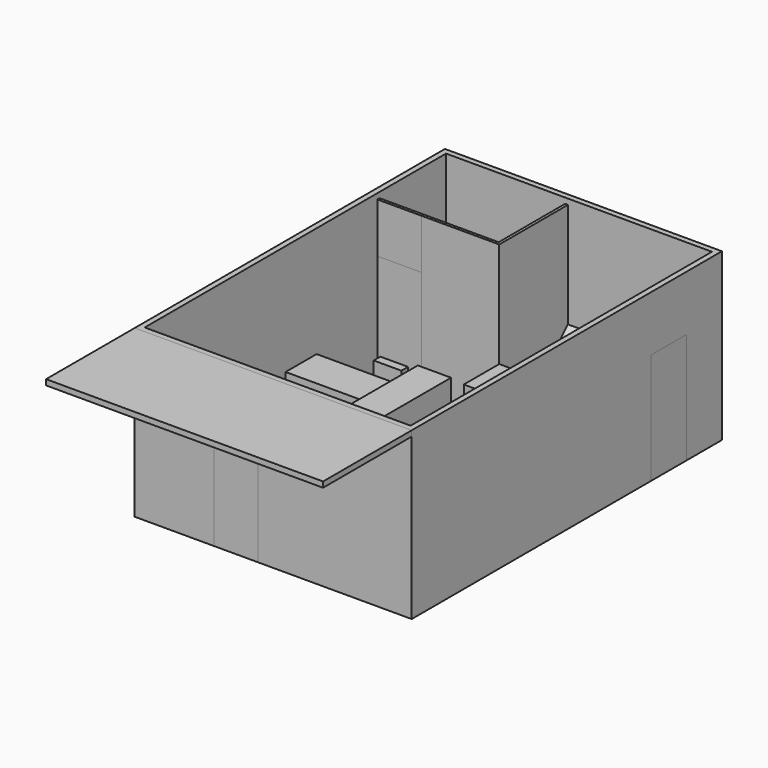
from build123d import *

# Parameters (mm, degrees)
F0_W      = 50
F0_H      = 70
F1_DEPTH  = 30
F2_T      = -1
F4_DEPTH  = 10
F3_W      = 4
F3_H      = 0.75
F3_W_2    = 5
F3_H_2    = 1.5
F3_H_3    = 5
F3_W_3    = 3
F3_H_4    = 3
F3_W_4    = 8.5
F3_H_5    = 3.5
F3_R      = 0.875
F5_DEPTH  = 6
F3_H_6    = 1.25
F3_H_7    = 18
F3_H_8    = 15
F6_DEPTH  = 20
F3_W_5    = 6.5
F3_W_6    = 0.2
F3_H_9    = 7
F3_H_10   = 8
F7_DEPTH  = 20
F8_DEPTH  = 10
F9_SIZE   = 9.99999
F10_DEPTH = 7
F12_DEPTH = 29
F3_W_7    = 8
F3_H_11   = 0.5
F13_DEPTH = 29
F14_DEPTH = 20
F15_DEPTH = 20
F16_W     = 50
F16_H     = 20
F17_DEPTH = 1
F18_W     = 8
F18_H     = 20
F19_DEPTH = 1
F20_DEPTH = 1
F21_W     = 8
F21_H     = 20
F22_DEPTH = 1
F23_DEPTH = 1


# Not quite as in the source:
# - a fillet or chamfer is up to 0.001 mm smaller than in the source, because OpenCascade refuses the exact size
# - the program builds the solid bodies; features that only make, move or delete a surface that nothing else refers to are left out


with BuildPart() as f1:
    # F0 (on Top) → F1 (new body)
    with BuildSketch(Plane.XY):
        Rectangle(F0_W, F0_H)
    extrude(amount=F1_DEPTH)

    # F2
    f2_openings = [f1.faces().sort_by_distance(p)[0] for p in [
        (0, 0, 30),
        (0, 0, 0),
    ]]
    offset(amount=F2_T, openings=f2_openings)

    # F3 (on Top) → F4, piece 5 (join)
    with BuildSketch(Plane.XY):
        with Locations((-15.5, 31.5)):
            Rectangle(F3_W, F3_H_3)
        with Locations((-15.5, 31)):
            Rectangle(F3_W_3, F3_H_4, mode=Mode.SUBTRACT)
        Polygon((-23, 34), (-23, 32), (-22.75, 32), (-18.75, 32), (-18.5, 32), (-18.5, 34), align=None)
        Polygon((-16.5, 4.8), (-24, 4.8), (-24, -2.2), (-4, -2.2), (-4, 4.8), (-11.5, 4.8), align=None)
        with Locations((13.25, 31.5)):
            Rectangle(F3_W_4, F3_H_3)
        with Locations((15, 31.25)):
            Rectangle(F3_W, F3_H_5, mode=Mode.SUBTRACT)
        with Locations((-21.5, -31.5)):
            Rectangle(F3_W_2, F3_H_3)
        Polygon((24, -9), (16, -9), (16, -10), (21, -10), (21, -28), (16, -28), (16, -29), (24, -29), align=None)
        with Locations((6.5, 31.5)):
            Rectangle(F3_W_2, F3_H_3)
        with Locations((5.25, 30.25)):
            Circle(F3_R, mode=Mode.SUBTRACT)
        with Locations((5.25, 32.75)):
            Circle(F3_R, mode=Mode.SUBTRACT)
        with Locations((7.75, 30.25)):
            Circle(F3_R, mode=Mode.SUBTRACT)
        with Locations((7.75, 32.75)):
            Circle(F3_R, mode=Mode.SUBTRACT)
    extrude(amount=F4_DEPTH)

    # F18 (on face) → F19 (cut)
    with BuildSketch(Plane.YZ.offset(25)):
        with Locations((23, 10)):
            Rectangle(F18_W, F18_H)
    extrude(amount=-F19_DEPTH, mode=Mode.SUBTRACT)

    # F21 (on face) → F22 (cut)
    with BuildSketch(Plane.XZ.offset(35)):
        with Locations((-6.7, 10)):
            Rectangle(F21_W, F21_H)
    extrude(amount=-F22_DEPTH, mode=Mode.SUBTRACT)


with BuildPart() as f4:
    # F3 (on Top) → F4 (new body)
    with BuildSketch(Plane.XY):
        Polygon((13, 18.5), (-2, 18.5), (-2, 10.5), (1, 10.5), (5, 10.5), (6, 10.5), (10, 10.5), (13, 10.5), align=None)
    extrude(amount=F4_DEPTH)


with BuildPart() as f4b:
    # F3 (on Top) → F4, piece 2 (new body)
    with BuildSketch(Plane.XY):
        with Locations((3, 8.875)):
            Rectangle(F3_W, F3_H)
    extrude(amount=F4_DEPTH)


with BuildPart() as f4c:
    # F3 (on Top) → F4, piece 3 (new body)
    with BuildSketch(Plane.XY):
        with Locations((8, 8.875)):
            Rectangle(F3_W, F3_H)
    extrude(amount=F4_DEPTH)


with BuildPart() as f4d:
    # F3 (on Top) → F4, piece 4 (new body)
    with BuildSketch(Plane.XY):
        with Locations((-14, 9.05)):
            Rectangle(F3_W_2, F3_H_2)
    extrude(amount=F4_DEPTH)


with BuildPart() as f5:
    # F3 (on Top) → F5 (new body)
    with BuildSketch(Plane.XY):
        with Locations((-14, 6.55)):
            Rectangle(F3_W_2, F3_H_5)
    extrude(amount=F5_DEPTH)


with BuildPart() as f5b:
    # F3 (on Top) → F5, piece 2 (new body)
    with BuildSketch(Plane.XY):
        with Locations((3, 9.875)):
            Rectangle(F3_W, F3_H_6)
    extrude(amount=F5_DEPTH)


with BuildPart() as f5c:
    # F3 (on Top) → F5, piece 3 (new body)
    with BuildSketch(Plane.XY):
        with Locations((8, 9.875)):
            Rectangle(F3_W, F3_H_6)
    extrude(amount=F5_DEPTH)


with BuildPart() as f5d:
    # F3 (on Top) → F5, piece 4 (new body)
    with BuildSketch(Plane.XY):
        with Locations((18.5, -19)):
            Rectangle(F3_W_2, F3_H_7)
    extrude(amount=F5_DEPTH)


with BuildPart() as f5e:
    # F3 (on Top) → F5, piece 5 (new body)
    with BuildSketch(Plane.XY):
        with Locations((9.3, -19)):
            Rectangle(F3_W, F3_H_8)
    extrude(amount=F5_DEPTH)


with BuildPart() as f5f:
    # F3 (on Top) → F5, piece 6 (new body)
    with BuildSketch(Plane.XY):
        Polygon((-3.7, -9.2), (-24, -9.2), (-24, -29), (-19, -29), (-3.7, -29), align=None)
    extrude(amount=F5_DEPTH)


with BuildPart() as f5g:
    # F3 (on Top) → F5, piece 7 (new body)
    with BuildSketch(Plane.XY):
        with BuildLine():
            Line((-18.75, 32), (-22.75, 32))
            Line((-22.75, 32), (-22.75, 29))
            ThreePointArc((-22.75, 29), (-20.75, 27), (-18.75, 29))
            Line((-18.75, 29), (-18.75, 32))
        make_face()
    extrude(amount=F5_DEPTH)


with BuildPart() as f6:
    # F3 (on Top) → F6 (new body)
    with BuildSketch(Plane.XY):
        Polygon((7.3, -26.5), (7.3, -11.5), (7.3, -4), (1.3, -4), (1.3, -34), (7.3, -34), align=None)
    extrude(amount=F6_DEPTH)


with BuildPart() as f6b:
    # F3 (on Top) → F6, piece 2 (new body)
    with BuildSketch(Plane.XY):
        with Locations((20.75, 31.5)):
            Rectangle(F3_W_5, F3_H_3)
    extrude(amount=F6_DEPTH)


with BuildPart() as f6c:
    # F3 (on Top) → F6, piece 3 (new body)
    with BuildSketch(Plane.XY):
        with Locations((-12.4, 22.5)):
            Rectangle(F3_W_6, F3_H_9)
    extrude(amount=F6_DEPTH)


with BuildPart() as f7:
    # F3 (on Top) → F7 (new body)
    with BuildSketch(Plane.XY):
        with Locations((-12.4, 30)):
            Rectangle(F3_W_6, F3_H_10)
    extrude(amount=F7_DEPTH)


with BuildPart() as f8:
    # F3 (on Top) → F8 (new body)
    with BuildSketch(Plane.XY):
        Polygon((4, 29), (4, 34), (-2, 34), (-2, 24), (4, 24), align=None)
    extrude(amount=F8_DEPTH)

    # F9 (size 10 in the source; OpenCascade refuses exactly that, so slightly less here)
    f9_edges = [f8.edges().sort_by_distance(p)[0] for p in [
        (1, 24, 10),
    ]]
    chamfer(f9_edges, length=F9_SIZE)


with BuildPart() as f10:
    # F3 (on Top) → F10 (new body)
    with BuildSketch(Plane.XY):
        with Locations((-15.5, 31)):
            Rectangle(F3_W_3, F3_H_4)
    extrude(amount=F10_DEPTH)


with BuildPart() as f10b:
    # F3 (on Top) → F10, piece 2 (new body)
    with BuildSketch(Plane.XY):
        with Locations((15, 31.25)):
            Rectangle(F3_W, F3_H_5)
    extrude(amount=F10_DEPTH)


with BuildPart() as f12:
    # F3 (on Top) → F12 (new body)
    with BuildSketch(Plane.XY):
        Polygon((-2, 24), (-2, 34), (-2.5, 34), (-2.5, 19), (-12.3, 19), (-12.5, 19), (-16, 19), (-16, 18.5), (-2, 18.5), align=None)
    extrude(amount=F12_DEPTH)


with BuildPart() as f13:
    # F3 (on Top) → F13 (new body)
    with BuildSketch(Plane.XY):
        with Locations((-20, 18.75)):
            Rectangle(F3_W_7, F3_H_11)
    extrude(amount=F13_DEPTH)

    # F3 (on Top) → F14 (cut)
    with BuildSketch(Plane.XY):
        with Locations((-20, 18.75)):
            Rectangle(F3_W_7, F3_H_11)
    extrude(amount=F14_DEPTH, mode=Mode.SUBTRACT)


with BuildPart() as f15:
    # F3 (on Top) → F15 (new body)
    with BuildSketch(Plane.XY):
        with Locations((-20, 18.75)):
            Rectangle(F3_W_7, F3_H_11)
    extrude(amount=F15_DEPTH)


with BuildPart() as f17:
    # F16 (on face) → F17 (new body)
    with BuildSketch(Plane.XY.offset(30)):
        with Locations((0, -45)):
            Rectangle(F16_W, F16_H)
    extrude(amount=-F17_DEPTH)


with BuildPart() as f20:
    # F18 (on face) → F20 (new body)
    with BuildSketch(Plane.YZ.offset(25)):
        with Locations((23, 10)):
            Rectangle(F18_W, F18_H)
    extrude(amount=-F20_DEPTH)


with BuildPart() as f23:
    # F21 (on face) → F23 (new body)
    with BuildSketch(Plane.XZ.offset(35)):
        with Locations((-6.7, 10)):
            Rectangle(F21_W, F21_H)
    extrude(amount=-F23_DEPTH)


solid = Compound([f1.part, f4.part, f4b.part, f4c.part, f4d.part, f5.part, f5b.part, f5c.part, f5d.part, f5e.part, f5f.part, f5g.part, f6.part, f6b.part, f6c.part, f7.part, f8.part, f10.part, f10b.part, f12.part, f13.part, f15.part, f17.part, f20.part, f23.part])
